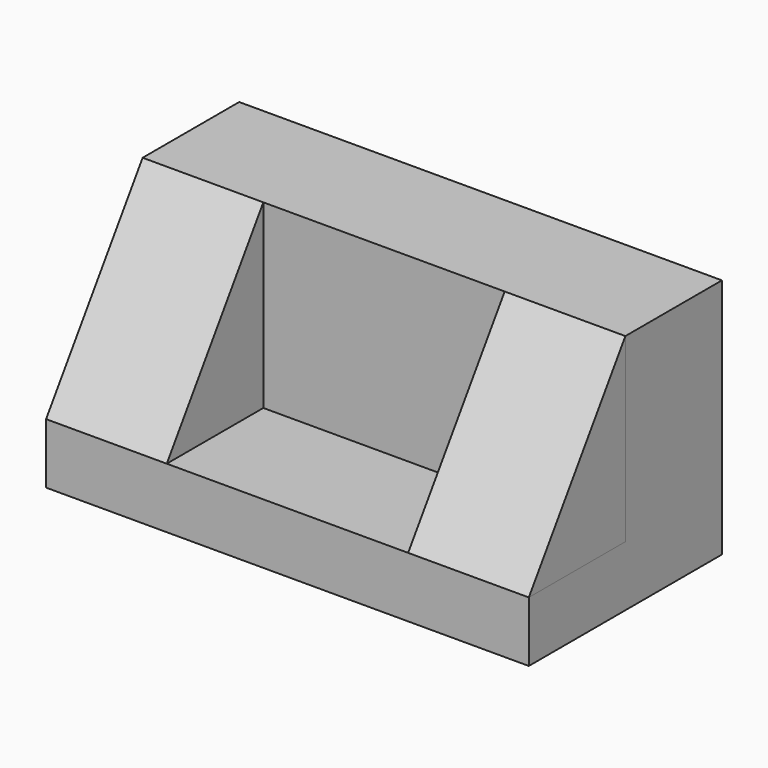
from build123d import *

# Parameters (mm, degrees)
F0_W     = 203.2
F0_H     = 101.6
F1_DEPTH = 50.8
F2_W     = 203.2
F2_H     = 25.4
F3_DEPTH = 50.8
F5_DEPTH = 50.8
F7_DEPTH = 50.8


# Not quite as in the source:
# - a feature names something its author has since deleted; it is built from what else it names


with BuildPart() as f1:
    # F0 (on Front) → F1 (new body)
    with BuildSketch(Plane.XZ):
        with Locations((-101.6, 50.8)):
            Rectangle(F0_W, F0_H)
    extrude(amount=F1_DEPTH)

    # F2 (on face) → F3 (join)
    with BuildSketch(Plane.XZ.offset(50.8)):
        with Locations((-101.6, 12.7)):
            Rectangle(F2_W, F2_H)
    extrude(amount=F3_DEPTH)


with BuildPart() as f5:
    # F4 (on face) → F5 (new body)
    with BuildSketch(Plane(origin=(-203.2, 0, 0), x_dir=(0, -1, 0), z_dir=(-1, 0, 0))):
        Polygon((101.6, 25.4), (50.8, 101.6), (50.8, 25.4), align=None)
    extrude(amount=-F5_DEPTH)


with BuildPart() as f7:
    # F6 (on face) → F7 (new body)
    with BuildSketch(Plane.YZ):
        Polygon((-50.8, 25.4), (-50.8, 101.6), (-101.6, 25.4), align=None)
    extrude(amount=-F7_DEPTH)


solid = Compound([f1.part, f5.part, f7.part])
